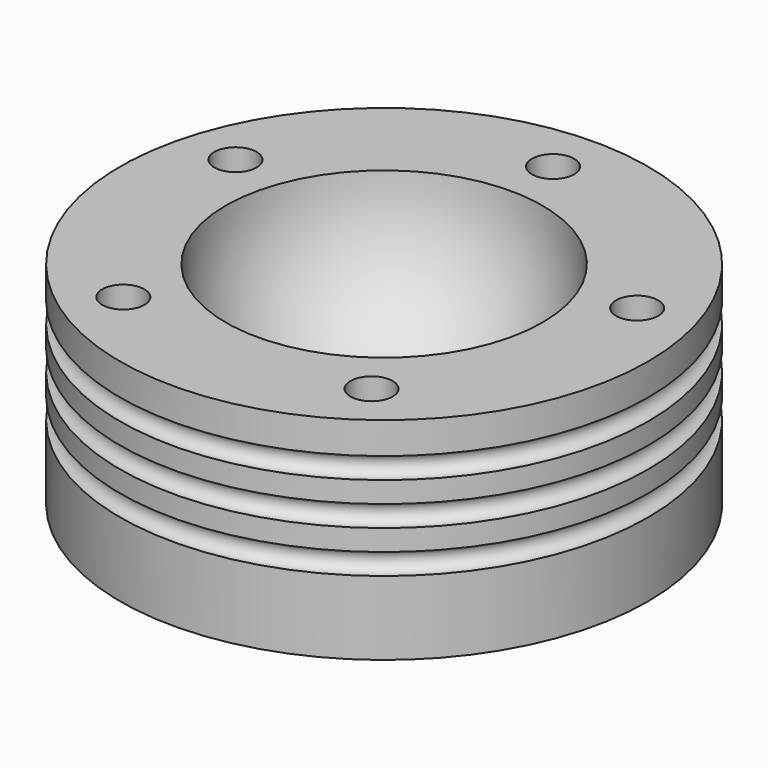
from build123d import *

# Parameters (mm, degrees)
F2_R     = 5
F3_DEPTH = 25


# Not quite as in the source:
# - a feature names something its author has since deleted; it is built from what else it names


with BuildPart() as f1:
    # F0 (on Front) → F1 (revolve)
    with BuildSketch(Plane.XZ):
        with BuildLine():
            Line((0, 12.5), (0, 0))
            Line((0, 0), (0, -5))
            Line((0, -5), (20, -5))
            Line((20, -5), (47.5, 0))
            Line((47.5, 0), (62.5, 0))
            Line((62.5, 0), (62.5, 17.5))
            ThreePointArc((62.5, 17.5), (60, 20), (62.5, 22.5))
            Line((62.5, 22.5), (62.5, 27.5))
            ThreePointArc((62.5, 27.5), (60, 30), (62.5, 32.5))
            Line((62.5, 32.5), (62.5, 37.5))
            ThreePointArc((62.5, 37.5), (60, 40), (62.5, 42.5))
            Line((62.5, 42.5), (62.5, 50))
            Line((62.5, 50), (37.5, 50))
            ThreePointArc((37.5, 50), (26.5165042945, 23.4834957055), (0, 12.5))
        make_face()
    revolve(axis=Axis((0, 0, 25), (0, 0, 1)))

    # F2 (on face) → F3 (cut)
    with BuildSketch(Plane.XY.offset(50)):
        with Locations((0, 50)):
            Circle(F2_R)
        with Locations((-47.5528258148, 15.4508497187)):
            Circle(F2_R)
        with Locations((-29.3892626146, -40.4508497187)):
            Circle(F2_R)
        with Locations((29.3892626146, -40.4508497187)):
            Circle(F2_R)
        with Locations((47.5528258148, 15.4508497187)):
            Circle(F2_R)
    extrude(amount=-F3_DEPTH, mode=Mode.SUBTRACT)


solid = f1.part
